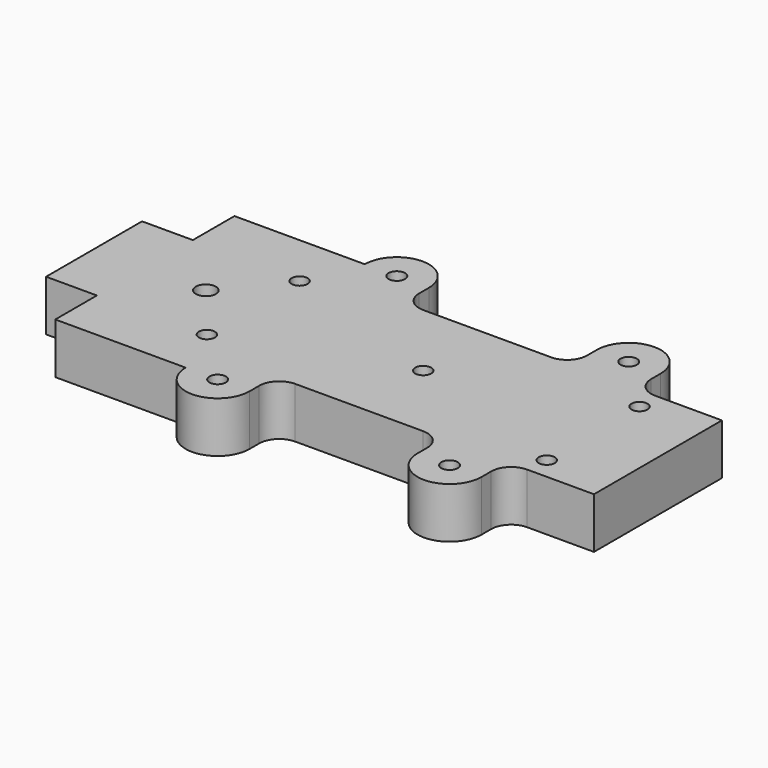
from build123d import *

# Parameters (mm, degrees)
F0_W           = 6.35
F0_H           = 15
F0_W_2         = 16.3
F0_H_2         = 4
F1_DEPTH       = 6.35
F2_D           = 2.05
F3_D           = 2.5
F4_R           = 2.5
F7_D           = 2.05
F7_DEPTH       = 6
F7_TIP         = 0.6158821345
F7_ON_F5_D     = 2.05
F7_ON_F5_DEPTH = 6
F7_ON_F5_TIP   = 0.6158821345
F8_D           = 2


# Not quite as in the source:
# - a length typed as a fraction of an inch, garbled in the dataset ("3 / 203.2 mm" for 3/8 in), is restored
# - a feature names something its author has since deleted; it is built from what else it names


with BuildPart() as f1:
    # F0 (on Top) → F1 (new body)
    with BuildSketch(Plane.XY):
        Polygon((-18.5, 10), (-34.8, 10), (-34.8, 7.5), (-34.8, -7.5), (-34.8, -10), (-18.5, -10), (-14.5, -10), (-11.8, -10), (-10.5, -10), (10.5, -10), (14.5, -10), (18.5, -10), (29.35, -10), (29.35, 10), (18.5, 10), (14.5000000137, 10), (10.5, 10), (-10.5, 10), (-14.5, 10), align=None)
        with Locations((-37.975, 0)):
            Rectangle(F0_W, F0_H)
        with BuildLine():
            Line((-18.5, 14), (-18.5, 10))
            Line((-18.5, 10), (-14.5, 10))
            ThreePointArc((-14.5, 10), (-17.3284271247, 11.1715728753), (-18.5, 14))
        make_face()
        with BuildLine():
            ThreePointArc((-10.5, 14), (-11.6715728753, 11.1715728753), (-14.5, 10))
            Line((-14.5, 10), (-10.5, 10))
            Line((-10.5, 10), (-10.5, 14))
        make_face()
        with BuildLine():
            ThreePointArc((-18.5, 14), (-17.3284271247, 11.1715728753), (-14.5, 10))
            ThreePointArc((-14.5, 10), (-11.6715728753, 11.1715728753), (-10.5, 14))
            Line((-10.5, 14), (-18.5, 14))
        make_face()
        with BuildLine():
            ThreePointArc((-10.5, 14), (-14.5, 18), (-18.5, 14))
            Line((-18.5, 14), (-10.5, 14))
        make_face()
        with BuildLine():
            Line((10.5, 14), (10.5, 10))
            Line((10.5, 10), (14.5000000137, 10))
            ThreePointArc((14.5000000137, 10), (11.6715728801, 11.1715728704), (10.5, 14))
        make_face()
        with BuildLine():
            ThreePointArc((10.5, 14), (11.6715728801, 11.1715728704), (14.5000000137, 10))
            ThreePointArc((14.5000000137, 10), (17.3284271296, 11.1715728801), (18.5, 14))
            ThreePointArc((18.5, 14), (14.5, 18), (10.5, 14))
        make_face()
        with BuildLine():
            ThreePointArc((18.5, 14), (17.3284271296, 11.1715728801), (14.5000000137, 10))
            Line((14.5000000137, 10), (18.5, 10))
            Line((18.5, 10), (18.5, 14))
        make_face()
        with BuildLine():
            ThreePointArc((18.5, -14), (17.3284271247, -11.1715728753), (14.5, -10))
            ThreePointArc((14.5, -10), (11.6715728753, -11.1715728753), (10.5, -14))
            ThreePointArc((10.5, -14), (14.5, -18), (18.5, -14))
        make_face()
        with BuildLine():
            Line((18.5, -14), (18.5, -10))
            Line((18.5, -10), (14.5, -10))
            ThreePointArc((14.5, -10), (17.3284271247, -11.1715728753), (18.5, -14))
        make_face()
        with BuildLine():
            Line((14.5, -10), (10.5, -10))
            Line((10.5, -10), (10.5, -14))
            ThreePointArc((10.5, -14), (11.6715728753, -11.1715728753), (14.5, -10))
        make_face()
        with BuildLine():
            ThreePointArc((-10.5, -14), (-11.6715728753, -11.1715728753), (-14.5, -10))
            ThreePointArc((-14.5, -10), (-17.3284271247, -11.1715728753), (-18.5, -14))
            ThreePointArc((-18.5, -14), (-14.5, -18), (-10.5, -14))
        make_face()
        with BuildLine():
            Line((-11.8, -10), (-14.5, -10))
            ThreePointArc((-14.5, -10), (-11.6715728753, -11.1715728753), (-10.5, -14))
            Line((-10.5, -14), (-10.5, -10))
            Line((-10.5, -10), (-11.8, -10))
        make_face()
        with BuildLine():
            Line((-14.5, -10), (-18.5, -10))
            Line((-18.5, -10), (-18.5, -14))
            ThreePointArc((-18.5, -14), (-17.3284271247, -11.1715728753), (-14.5, -10))
        make_face()
        with Locations((-26.65, 12)):
            Rectangle(F0_W_2, F0_H_2)
        with Locations((-26.65, -12)):
            Rectangle(F0_W_2, F0_H_2)
    extrude(amount=F1_DEPTH)

    # F2 (through all)
    with Locations(Plane(origin=(0, 0, 0), x_dir=(1, 0, 0), z_dir=(0, 0, -1))):
        with Locations((-14.5, -14), (14.5, -14), (14.5, 14), (-14.5, 14)):
            Hole(F2_D / 2)

    # F3 (through all)
    with Locations(Plane(origin=(0, 0, 0), x_dir=(1, 0, 0), z_dir=(0, 0, -1))):
        with Locations((-27.175, 0)):
            Hole(F3_D / 2)

    # F4
    f4_edges = [f1.edges().sort_by_distance(p)[0] for p in [
        (-10.5, 10, 3.175),
        (10.5, 10, 3.175),
        (18.5, 10, 3.175),
        (-10.5, -10, 3.175),
        (10.5, -10, 3.175),
        (18.5, -10, 3.175),
        (-10.5, 14, 3.175),
    ]]
    fillet(f4_edges, radius=F4_R)

    # F7
    with Locations(Plane(origin=(-34.8, 0, 0), x_dir=(0, -1, 0), z_dir=(-1, 0, 0))):
        with Locations((-11.25, 3.175)):
            Hole(F7_D / 2, depth=F7_DEPTH)
            with Locations((0, 0, -(F7_DEPTH + F7_TIP / 2))):  # 118° drill point
                Cone(0, F7_D / 2, F7_TIP, mode=Mode.SUBTRACT)

    # F7 on F5
    with Locations(Plane(origin=(-34.8, 0, 0), x_dir=(0, -1, 0), z_dir=(-1, 0, 0))):
        with Locations((11.25, 3.175)):
            Hole(F7_ON_F5_D / 2, depth=F7_ON_F5_DEPTH)
            with Locations((0, 0, -(F7_ON_F5_DEPTH + F7_ON_F5_TIP / 2))):  # 118° drill point
                Cone(0, F7_ON_F5_D / 2, F7_ON_F5_TIP, mode=Mode.SUBTRACT)

    # F8 (through all)
    with Locations(Plane(origin=(0, 0, 0), x_dir=(1, 0, 0), z_dir=(0, 0, -1))):
        with Locations((-21.25, -7.25), (-21.25, 7.25), (0, 0), (21.25, -7.25), (21.25, 7.25)):
            Hole(F8_D / 2)


solid = f1.part
